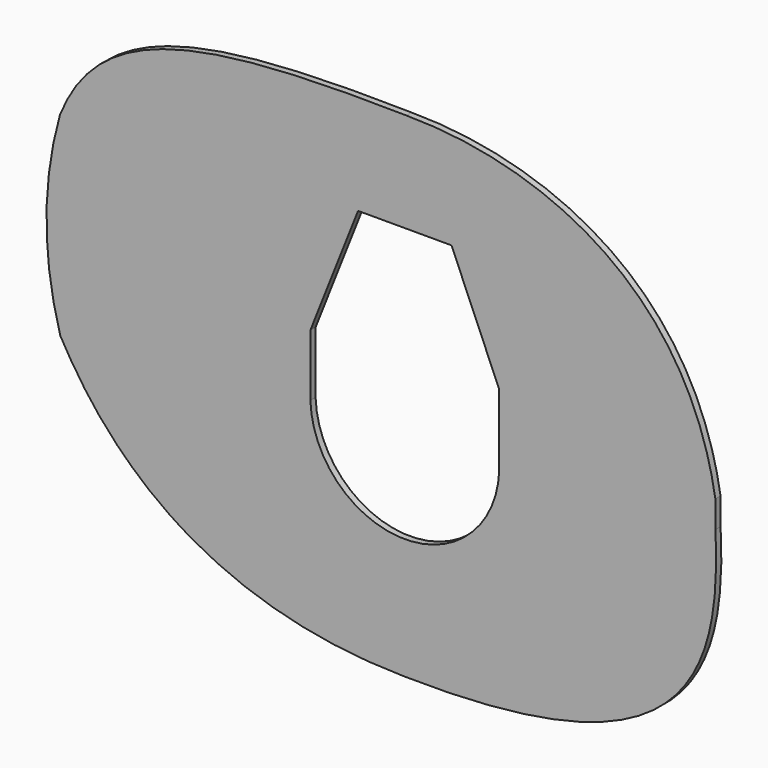
from build123d import *

# Parameters (mm, degrees)
F1_DEPTH = 2


with BuildPart() as f1:
    # F0 (on Front) → F1 (new body)
    with BuildSketch(Plane.XZ):
        with BuildLine():
            Line((-124.6721289065, 66.9943112569), (-124.6721289065, -3.1820335149))
            add(Edge.make_bspline(
                [(-108.7886020541, -16.6170091142), (-115.0603290285, -12.3232285742), (-120.2999981868, -7.7183339998), (-124.6721289065, -3.1820335149)],
                knots=[0.4585261262, 0.4585261262, 0.4585261262, 0.4585261262, 0.6354781501, 0.6354781501, 0.6354781501, 0.6354781501], degree=3))
            Line((-108.7886020541, -16.6170091142), (-108.7886020541, 66.9943112569))
            Line((-108.7886020541, 66.9943112569), (-124.6721289065, 66.9943112569))
        make_face()
        with BuildLine():
            add(Edge.make_bspline(
                [(-142.2094079373, 80.4314068878), (-130.2931281445, 110.3476141939), (-98.2848527548, 116.0134827146), (-35.7470019427, 114.8680118272)],
                knots=[0, 0, 0, 0, 1, 1, 1, 1], degree=3))
            ThreePointArc((-142.2094079373, 80.4314068878), (-146.3504948166, 50.5368703201), (-142.0856537936, 20.6597377906))
            add(Edge.make_bspline(
                [(-124.6721289065, -3.1820335149), (-133.6787350082, 6.1627629347), (-139.0038412424, 15.2164724191), (-142.0856537936, 20.6597377906)],
                knots=[0.6354781501, 0.6354781501, 0.6354781501, 0.6354781501, 1, 1, 1, 1], degree=3))
            Line((-124.6721289065, -3.1820335149), (-124.6721289065, 66.9943112569))
            Line((-124.6721289065, 66.9943112569), (-108.7886020541, 66.9943112569))
            Line((-108.7886020541, 66.9943112569), (-108.7886020541, -16.6170091142))
            add(Edge.make_bspline(
                [(-36.381947872, -37.122189497), (-69.3556272485, -36.7804960017), (-92.5370180869, -27.743248389), (-108.7886020541, -16.6170091142)],
                knots=[0, 0, 0, 0, 0.4585261262, 0.4585261262, 0.4585261262, 0.4585261262], degree=3))
            add(Edge.make_bspline(
                [(-36.381947872, -37.122189497), (47.0810634374, -38.6126036396), (61.6125640752, -9.5495949141), (59.2237142208, 33.6754252563)],
                knots=[0, 0, 0, 0, 1, 1, 1, 1], degree=3))
            Line((59.2237142208, 33.6754252563), (59.2237142208, 42.0407210837))
            add(Edge.make_bspline(
                [(-35.7470019427, 114.8680118272), (4.2317536953, 114.8997140476), (50.434487808, 96.2695801058), (59.2237142208, 42.0407210837)],
                knots=[0, 0, 0, 0, 1, 1, 1, 1], degree=3))
        make_face()
        with BuildLine():
            Line((-65.2386816857, 47.185676674), (-50.5756217741, 84.2391779074))
            Line((-50.5756217741, 84.2391779074), (-21.8579741833, 84.2391779074))
            Line((-21.8579741833, 84.2391779074), (-7.197354984, 50.0167762288))
            Line((-7.197354984, 50.0167762288), (-7.197354984, 28.1597529901))
            ThreePointArc((-7.197354984, 28.1597529901), (-36.2556737781, 0.0750783929), (-65.2386816857, 28.237466271))
            Line((-65.2386816857, 28.237466271), (-65.2386816857, 47.185676674))
        make_face(mode=Mode.SUBTRACT)
    extrude(amount=F1_DEPTH)


solid = f1.part
